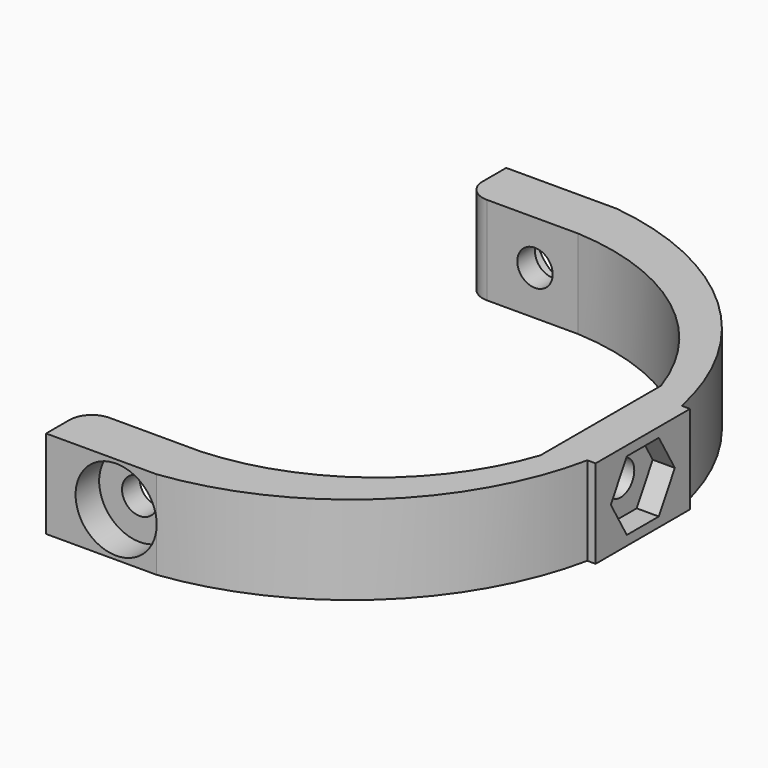
from build123d import *

# Parameters (mm, degrees)
F0_W          = 11
F0_H          = 4
F1_DEPTH      = 6
F1_DEPTH_BACK = 6
F2_R          = 5.5
F2_R_2        = 2.4
F3_DEPTH      = 4
F4_DEPTH      = 10.8
F5_R          = 2.4
F6_DEPTH      = 4
F7_DEPTH      = 10
F8_R          = 2.3
F9_DEPTH      = 3
F10_DEPTH     = 14


# Not quite as in the source:
# - a feature names something its author has since deleted; it is built from what else it names


with BuildPart() as f1:
    # F0 (on Top) → F1 (new body, two sides)
    with BuildSketch(Plane.XY) as f1_sk:
        with Locations((0, 37)):
            Rectangle(F0_W, F0_H)
        with BuildLine():
            ThreePointArc((-9.5, 35), (-8.6213203436, 32.8786796564), (-6.5, 32))
            Line((-6.5, 32), (5.8594679956, 32))
            ThreePointArc((5.8594679956, 32), (23.5324507486, 25.5063318649), (34.5083337044, 10.2082261463))
            Line((34.5083337044, 10.2082261463), (34.5083337044, -10.2082261463))
            ThreePointArc((34.5083337044, -10.2082261463), (23.5324507486, -25.5063318649), (5.8594679956, -32))
            Line((5.8594679956, -32), (-6.5, -32))
            ThreePointArc((-6.5, -32), (-8.6213203436, -32.8786796564), (-9.5, -35))
            Line((-9.5, -35), (-9.5, -39))
            Line((-9.5, -39), (-5.5, -39))
            Line((-5.5, -39), (-5.5, -35))
            Line((-5.5, -35), (5.5, -35))
            Line((5.5, -35), (5.5, -39))
            ThreePointArc((5.5, -39), (27.2702801405, -28.8873683489), (39.0994077402, -8))
            Line((39.0994077402, -8), (40.2236692607, -8))
            Line((40.2236692607, -8), (40.2236692607, 8))
            Line((40.2236692607, 8), (39.0994077402, 8))
            ThreePointArc((39.0994077402, 8), (27.2702801405, 28.8873683489), (5.5, 39))
            Line((5.5, 39), (5.5, 35))
            Line((5.5, 35), (-5.5, 35))
            Line((-5.5, 35), (-5.5, 39))
            Line((-5.5, 39), (-9.5, 39))
            Line((-9.5, 39), (-9.5, 35))
        make_face()
        with Locations((0, -37)):
            Rectangle(F0_W, F0_H)
    extrude(amount=F1_DEPTH)
    extrude(f1_sk.sketch, amount=-F1_DEPTH_BACK)

    # F2 (on face) → F3 (cut)
    with BuildSketch(Plane.XZ.offset(39)):
        Circle(F2_R)
        Circle(F2_R_2, mode=Mode.SUBTRACT)
    extrude(amount=-F3_DEPTH, mode=Mode.SUBTRACT)

    # F4 (cut): a face of the model
    f4_faces = [f1.faces().sort_by_distance(p)[0] for p in [
        (0, -39, 0),
    ]]
    extrude(f4_faces, amount=-F4_DEPTH, mode=Mode.SUBTRACT)

    # F5 (on face) → F6 (cut)
    with BuildSketch(Plane(origin=(0, 39, 0), x_dir=(-1, 0, 0), z_dir=(0, 1, 0))):
        with BuildLine():
            ThreePointArc((-5.5, 3.96e-08), (-1.98e-08, -5.5), (5.5, 0))
            ThreePointArc((5.5, 0), (1.98e-08, 5.5), (-5.5, 3.96e-08))
        make_face()
        Circle(F5_R, mode=Mode.SUBTRACT)
    extrude(amount=-F6_DEPTH, mode=Mode.SUBTRACT)

    # F7 (cut): a face of the model
    f7_faces = [f1.faces().sort_by_distance(p)[0] for p in [
        (0, 39, 0),
    ]]
    extrude(f7_faces, amount=-F7_DEPTH, mode=Mode.SUBTRACT)

    # F8 (on face) → F9 (cut)
    with BuildSketch(Plane.YZ.offset(40.2236692607)):
        Polygon((2.7135462652, -4.7), (5.4270925304, 0), (2.7135462652, 4.7), (-2.7135462652, 4.7), (-5.4270925304, 0), (-2.7135462652, -4.7), align=None)
        Circle(F8_R, mode=Mode.SUBTRACT)
    extrude(amount=-F9_DEPTH, mode=Mode.SUBTRACT)

    # F10 (cut): a face of the model
    f10_faces = [f1.faces().sort_by_distance(p)[0] for p in [
        (40.2236692607, 0, 0),
    ]]
    extrude(f10_faces, amount=-F10_DEPTH, mode=Mode.SUBTRACT)


solid = f1.part
